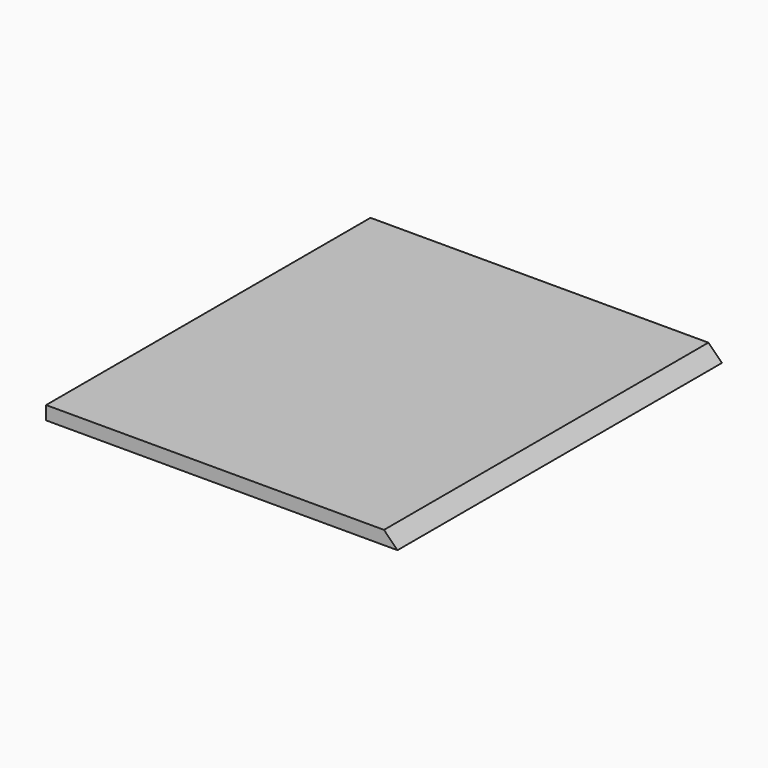
from build123d import *

# Parameters (mm, degrees)
F0_W     = 660.4
F0_H     = 762
F1_DEPTH = 25.4
F2_SIZE  = 25.39999


# Not quite as in the source:
# - a fillet or chamfer is up to 0.001 mm smaller than in the source, because OpenCascade refuses the exact size


with BuildPart() as f1:
    # F0 (on Top) → F1 (new body)
    with BuildSketch(Plane.XY):
        with Locations((-148.2397035837, -222.647351265)):
            Rectangle(F0_W, F0_H)
    extrude(amount=F1_DEPTH)

    # F2 (size 25.4 in the source; OpenCascade refuses exactly that, so slightly less here)
    f2_edges = [f1.edges().sort_by_distance(p)[0] for p in [
        (181.960296, -222.647351, 25.4),
    ]]
    chamfer(f2_edges, length=F2_SIZE)


solid = f1.part
